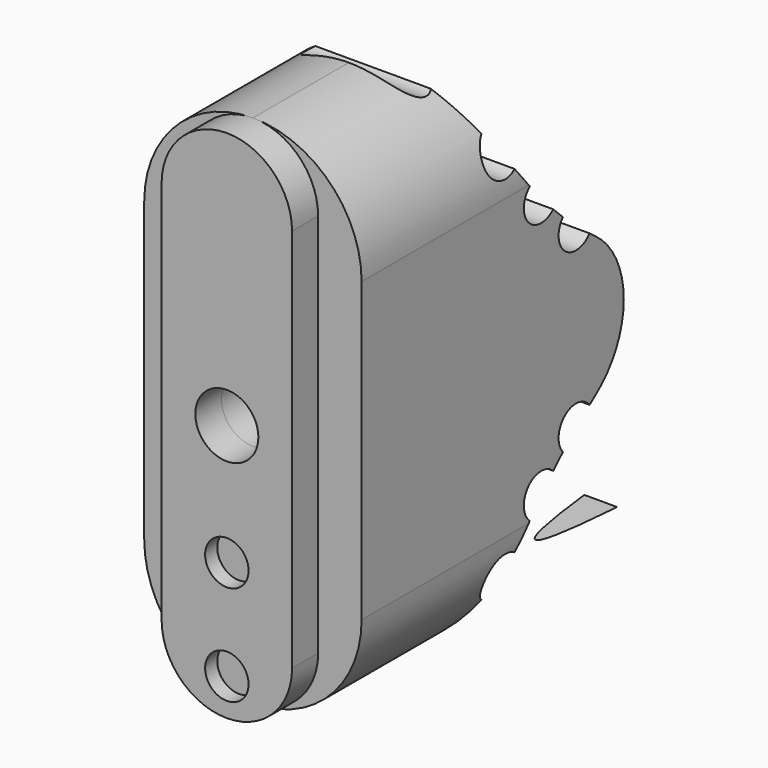
from build123d import *
from build123d import SkipClean  # not in build123d's __all__

# Parameters (mm, degrees)
F1_DEPTH = 1.905
F2_R     = 1.27
F3_DEPTH = 0.889
F2_R_2   = 1.8415
F4_DEPTH = 25.4
F5_R     = 1.8415
F6_DEPTH = 25.4
F8_DEPTH = 25.4


# Not quite as in the source:
# - after a boolean that leaves OpenCascade's solid faulty, fix() repairs it


with BuildPart() as f1:
    # F0 (on Front) → F1 (new body)
    with BuildSketch(Plane.XZ):
        with BuildLine():
            Line((-3.81, 22.479), (-3.81, 0))
            ThreePointArc((-3.81, 0), (0, -3.81), (3.81, 0))
            Line((3.81, 0), (3.81, 22.479))
            ThreePointArc((3.81, 22.479), (0, 26.289), (-3.81, 22.479))
        make_face()
    extrude(amount=F1_DEPTH)

    # F2 (on face) → F3 (cut)
    with BuildSketch(Plane.XZ.offset(1.905)):
        with Locations((0, 4.191)):
            Circle(F2_R)
        with Locations((0, -1.651)):
            Circle(F2_R)
    extrude(amount=-F3_DEPTH, mode=Mode.SUBTRACT)

    # F2 (on face) → F4 (cut)
    with BuildSketch(Plane.XZ.offset(1.905)):
        with Locations((0, 11.2395)):
            Circle(F2_R_2)
    extrude(amount=-F4_DEPTH, mode=Mode.SUBTRACT)

    # F5 (on face) → F6 (join)
    with BuildSketch(Plane(origin=(0, 0, 0), x_dir=(-1, 0, 0), z_dir=(0, 1, 0))):
        with BuildLine():
            Line((6.35, 2.54), (6.35, 19.939))
            ThreePointArc((6.35, 19.939), (4.4901280605, 24.4291280605), (0, 26.289))
            ThreePointArc((0, 26.289), (2.6940768363, 25.1730768363), (3.81, 22.479))
            Line((3.81, 22.479), (3.81, 0))
            ThreePointArc((3.81, 0), (2.6940768283, -2.6940768443), (-2.26e-08, -3.81))
            ThreePointArc((-2.26e-08, -3.81), (4.4901280526, -1.9501280685), (6.35, 2.54))
        make_face()
        with BuildLine():
            ThreePointArc((3.81, 22.479), (2.6940768363, 25.1730768363), (0, 26.289))
            ThreePointArc((0, 26.289), (-2.6940768363, 25.1730768363), (-3.81, 22.479))
            Line((-3.81, 22.479), (-3.81, 0))
            ThreePointArc((-3.81, 0), (-2.6940768443, -2.6940768283), (-2.26e-08, -3.81))
            ThreePointArc((-2.26e-08, -3.81), (2.6940768283, -2.6940768443), (3.81, 0))
            Line((3.81, 0), (3.81, 22.479))
        make_face()
        with Locations((0, 11.2395)):
            Circle(F5_R, mode=Mode.SUBTRACT)
        with BuildLine():
            ThreePointArc((-3.81, 22.479), (-2.6940768363, 25.1730768363), (0, 26.289))
            ThreePointArc((0, 26.289), (-4.4901280605, 24.4291280605), (-6.35, 19.939))
            Line((-6.35, 19.939), (-6.35, 2.54))
            ThreePointArc((-6.35, 2.54), (-4.4901280685, -1.9501280526), (-2.26e-08, -3.81))
            ThreePointArc((-2.26e-08, -3.81), (-2.6940768443, -2.6940768283), (-3.81, 0))
            Line((-3.81, 0), (-3.81, 22.479))
        make_face()
    with SkipClean():  # cleaning this boolean's faces spoils the solid; the shape is the same uncleaned
        extrude(amount=F6_DEPTH)

    # F7 (on face) → F8 (cut)
    with BuildSketch(Plane(origin=(-6.35, 0, 0), x_dir=(0, -1, 0), z_dir=(-1, 0, 0))):
        with BuildLine():
            Line((-25.4, 19.939), (-12.2053374914, 19.939))
            ThreePointArc((-12.2053374914, 19.939), (-11.7457258145, 20.5152553369), (-11.302214531, 21.1039919914))
            ThreePointArc((-11.302214531, 21.1039919914), (-9.5173742951, 21.4459716607), (-9.9017532138, 23.2221635447))
            ThreePointArc((-9.9017532138, 23.2221635447), (-9.3158304407, 24.2593417985), (-8.7768069595, 25.3216496223))
            ThreePointArc((-8.7768069595, 25.3216496223), (-7.181162456, 27.1575655787), (-9.5247212955, 26.5061051072))
            Line((-9.5247212955, 26.5061051072), (-25.4, 26.8387477845))
            Line((-25.4, 26.8387477845), (-25.4, 19.939))
        make_face()
        with BuildLine():
            ThreePointArc((-17.0665918725, 7.1409536759), (-19.1452058545, 11.2395), (-17.0665918725, 15.3380463241))
            ThreePointArc((-17.0665918725, 15.3380463241), (-16.856462314, 15.4935129075), (-16.647866537, 15.6510314514))
            ThreePointArc((-16.647866537, 15.6510314514), (-14.839279057, 15.4732223146), (-14.7045819334, 17.2855306346))
            ThreePointArc((-14.7045819334, 17.2855306346), (-14.3464292382, 17.6233283273), (-13.9945729627, 17.9676795951))
            ThreePointArc((-13.9945729627, 17.9676795951), (-12.1783266761, 18.0297617042), (-12.2836351449, 19.8440149633))
            ThreePointArc((-12.2836351449, 19.8440149633), (-12.2444315173, 19.8914623085), (-12.2053374914, 19.939))
            Line((-12.2053374914, 19.939), (-25.4, 19.939))
            Line((-25.4, 19.939), (-25.4, 2.54))
            Line((-25.4, 2.54), (-12.2053374914, 2.54))
            ThreePointArc((-12.2053374914, 2.54), (-12.2444315173, 2.5875376915), (-12.2836351449, 2.6349850367))
            ThreePointArc((-12.2836351449, 2.6349850367), (-12.1783266761, 4.4492382958), (-13.9945729627, 4.5113204049))
            ThreePointArc((-13.9945729627, 4.5113204049), (-14.3464292382, 4.8556716727), (-14.7045819334, 5.1934693654))
            ThreePointArc((-14.7045819334, 5.1934693654), (-14.839279057, 7.0057776854), (-16.647866537, 6.8279685486))
            ThreePointArc((-16.647866537, 6.8279685486), (-16.856462314, 6.9854870925), (-17.0665918725, 7.1409536759))
        make_face()
        with BuildLine():
            ThreePointArc((-11.302214531, 1.3750080086), (-11.7457258145, 1.9637446631), (-12.2053374914, 2.54))
            Line((-12.2053374914, 2.54), (-25.4, 2.54))
            Line((-25.4, 2.54), (-25.4, -3.7370298523))
            Line((-25.4, -3.7370298523), (-9.5248500713, -3.9809859967))
            ThreePointArc((-9.5248500713, -3.9809859967), (-7.193651257, -4.6979516798), (-8.7768069595, -2.8426496223))
            ThreePointArc((-8.7768069595, -2.8426496223), (-9.3158304407, -1.7803417985), (-9.9017532138, -0.7431635447))
            ThreePointArc((-9.9017532138, -0.7431635447), (-9.5173742951, 1.0330283393), (-11.302214531, 1.3750080086))
        make_face()
    extrude(amount=-F8_DEPTH, mode=Mode.SUBTRACT)

    add(f1.part.fix(), mode=Mode.REPLACE)


solid = f1.part
